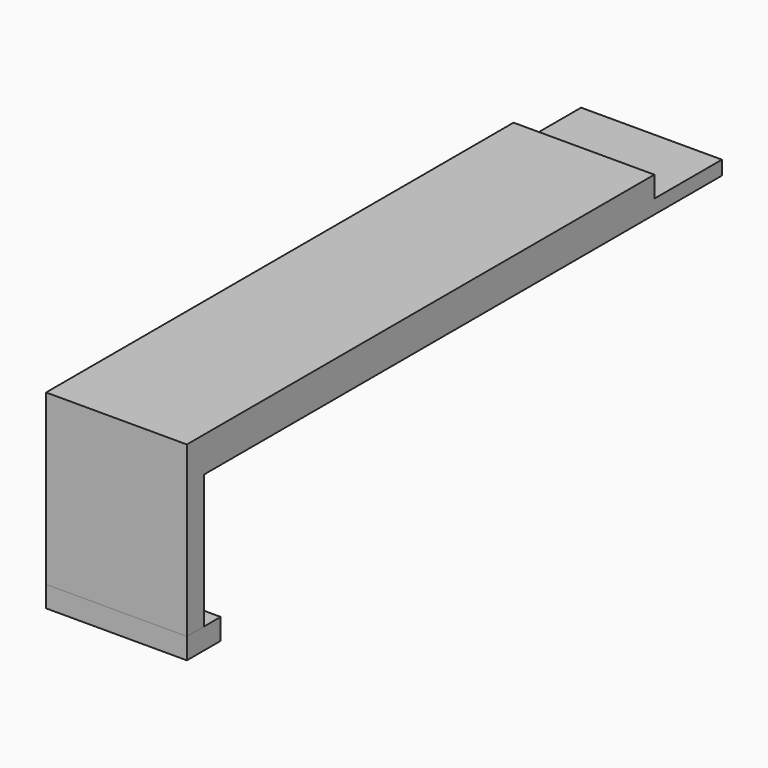
from build123d import *

# Parameters (mm, degrees)
F0_W     = 20
F0_H     = 3
F1_DEPTH = 24
F2_DEPTH = 3
F0_H_2   = 77
F0_H_3   = 12
F4_DEPTH = 5
F5_DEPTH = 3


with BuildPart() as f1:
    # F0 (on Top) → F1 (new body)
    with BuildSketch(Plane.XY):
        with Locations((0, -46)):
            Rectangle(F0_W, F0_H)
    extrude(amount=-F1_DEPTH)

    # F0 (on Top) → F4 (join)
    with BuildSketch(Plane.XY):
        with Locations((0, -43)):
            Rectangle(F0_W, F0_H)
        with Locations((0, -3)):
            Rectangle(F0_W, F0_H_2)
        with Locations((0, 41.5)):
            Rectangle(F0_W, F0_H_3)
    extrude(amount=-F4_DEPTH)

    # F0 (on Top) → F5 (cut)
    with BuildSketch(Plane.XY):
        with Locations((0, 41.5)):
            Rectangle(F0_W, F0_H_3)
    extrude(amount=-F5_DEPTH, mode=Mode.SUBTRACT)


with BuildPart() as f2:
    # F0 (on Top) → F2 (new body)
    with BuildSketch(Plane.XY):
        with Locations((0, -43)):
            Rectangle(F0_W, F0_H)
        with Locations((0, -46)):
            Rectangle(F0_W, F0_H)
    extrude(amount=-F2_DEPTH)


with BuildPart() as f2_1:
    # F3: moved
    add(f2.part.moved(Location((0, 0, -24))))


solid = Compound([f1.part, f2_1.part])
